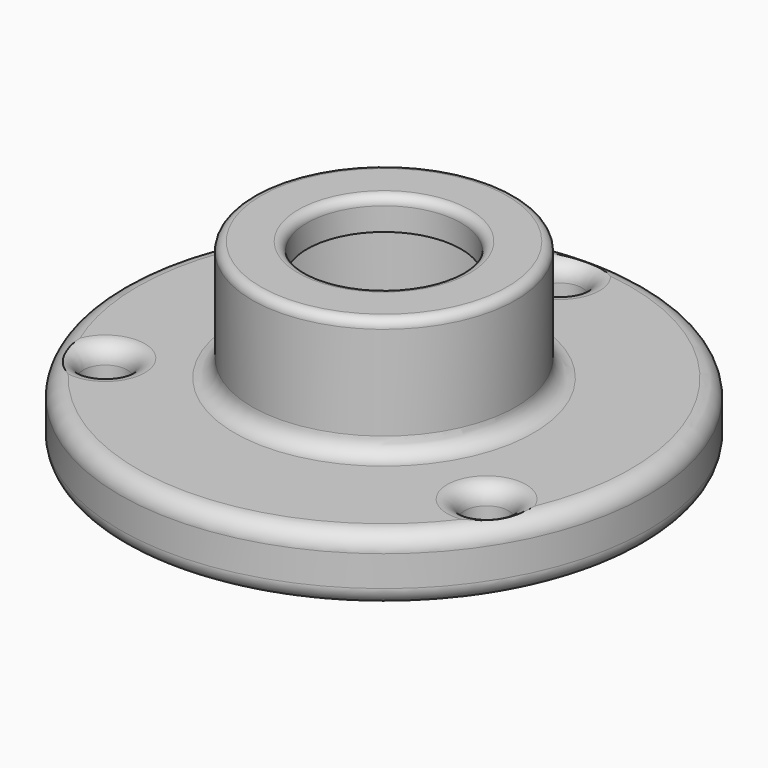
from build123d import *

# Parameters (mm, degrees)
F0_W     = 38.1
F0_H     = 34.6730154096
F2_R     = 6.35
F3_DEPTH = 18.9502071143
F4_R     = 31.75
F5_DEPTH = 44.45
F6_R     = 22.225
F7_DEPTH = 25.4
F8_R     = 2.54


# Not quite as in the source:
# - a fillet or chamfer that OpenCascade refuses, or shapes differently, is made with other operations: its cross-section is extruded or revolved along the edge and cut away or added


with BuildPart() as f1:
    # F0 (on Front) → F1 (revolve)
    with BuildSketch(Plane.XZ):
        Polygon((-76.2, 0), (0, 0), (0, 18.9492071143), (-38.1, 18.9492071143), (-76.2, 18.9492071143), align=None)
        with Locations((-19.05, 36.2857148192)):
            Rectangle(F0_W, F0_H)
    revolve(axis=Axis((0, 0, 36.2857148192), (0, 0, -1)))

    # F2 (on face) → F3 (cut, through all)
    with BuildSketch(Plane.XY.offset(18.9492071143)):
        with Locations((-54.9926131403, -31.75)):
            Circle(F2_R)
        with Locations((54.9926131403, -31.75)):
            Circle(F2_R)
        with Locations((0, 63.5)):
            Circle(F2_R)
    extrude(amount=-F3_DEPTH, mode=Mode.SUBTRACT)

    # F4 (on face) → F5 (cut)
    with BuildSketch(Plane(origin=(0, 0, 0), x_dir=(1, 0, 0), z_dir=(0, 0, -1))):
        Circle(F4_R)
    extrude(amount=-F5_DEPTH, mode=Mode.SUBTRACT)

    # F6 (on face) → F7 (cut)
    with BuildSketch(Plane.XY.offset(53.622222524)):
        Circle(F6_R)
    extrude(amount=-F7_DEPTH, mode=Mode.SUBTRACT)

    # F8
    f8_edges = [f1.edges().sort_by_distance(p)[0] for p in [
        (38.1, 0, 53.622223),
        (-22.225, 0, 53.622223),
    ]]
    fillet(f8_edges, radius=F8_R)

    # F9: fillet of radius 5.08 on 5 edges, made by hand

    # F9_s1 → F9_t2 (revolve)
    with BuildSketch(Plane.XZ):
        with BuildLine():
            ThreePointArc((-38.0996, 24.0301727998), (-39.5878975516, 20.4371046659), (-43.1809656854, 18.9488071143))
            Line((-43.1809656854, 18.9488071143), (-43.1809656854, 18.4406705458))
            ThreePointArc((-43.1809656854, 18.4406705458), (-40.6404828427, 18.4410705458), (-38.1, 18.4410705458))
            Line((-38.1, 18.4410705458), (-37.5918634315, 18.9492071143))
            ThreePointArc((-37.5918634315, 18.9492071143), (-37.5918634315, 21.489689957), (-37.5914634315, 24.0301727998))
            Line((-37.5914634315, 24.0301727998), (-38.0996, 24.0301727998))
        make_face()
    revolve(axis=Axis((0, 0, 18.9492071143), (0, 0, -1)))

    # F9_s3 → F9_t4 (revolve, cut)
    with BuildSketch(Plane.XZ):
        with BuildLine():
            ThreePointArc((-71.1190343146, 18.9496071143), (-74.7121024484, 17.4613095628), (-76.2004, 13.8682414289))
            Line((-76.2004, 13.8682414289), (-76.7085365685, 13.8682414289))
            ThreePointArc((-76.7085365685, 13.8682414289), (-76.7081365685, 16.4087242716), (-76.7081365685, 18.9492071143))
            Line((-76.7081365685, 18.9492071143), (-76.2, 19.4573436829))
            ThreePointArc((-76.2, 19.4573436829), (-73.6595171573, 19.4573436829), (-71.1190343146, 19.4577436829))
            Line((-71.1190343146, 19.4577436829), (-71.1190343146, 18.9496071143))
        make_face()
    revolve(axis=Axis((0, 0, 18.9492071143), (0, 0, -1)), mode=Mode.SUBTRACT)

    # F9_s5 → F9_t6 (revolve, cut)
    with BuildSketch(Plane.XZ.offset(31.75)):
        with BuildLine():
            ThreePointArc((-43.5616474549, 18.9496071143), (-47.1547155887, 17.4613095628), (-48.6430131403, 13.8682414289))
            Line((-48.6430131403, 13.8682414289), (-49.1511497089, 13.8682414289))
            ThreePointArc((-49.1511497089, 13.8682414289), (-49.1507497089, 16.4087242716), (-49.1507497089, 18.9492071143))
            Line((-49.1507497089, 18.9492071143), (-48.6426131403, 19.4573436829))
            ThreePointArc((-48.6426131403, 19.4573436829), (-46.1021302976, 19.4573436829), (-43.5616474549, 19.4577436829))
            Line((-43.5616474549, 19.4577436829), (-43.5616474549, 18.9496071143))
        make_face()
    revolve(axis=Axis((-54.9926131403, -31.75, 18.9492071143), (0, 0, 1)), mode=Mode.SUBTRACT)

    # F9_s7 → F9_t8 (revolve, cut)
    with BuildSketch(Plane.XZ.offset(31.75)):
        with BuildLine():
            ThreePointArc((66.4235788257, 18.9496071143), (62.8305106919, 17.4613095628), (61.3422131403, 13.8682414289))
            Line((61.3422131403, 13.8682414289), (60.8340765718, 13.8682414289))
            ThreePointArc((60.8340765718, 13.8682414289), (60.8344765718, 16.4087242716), (60.8344765718, 18.9492071143))
            Line((60.8344765718, 18.9492071143), (61.3426131403, 19.4573436829))
            ThreePointArc((61.3426131403, 19.4573436829), (63.883095983, 19.4573436829), (66.4235788257, 19.4577436829))
            Line((66.4235788257, 19.4577436829), (66.4235788257, 18.9496071143))
        make_face()
    revolve(axis=Axis((54.9926131403, -31.75, 18.9492071143), (0, 0, 1)), mode=Mode.SUBTRACT)

    # F9_s9 → F9_t10 (revolve, cut)
    with BuildSketch(Plane.XZ.offset(-63.5)):
        with BuildLine():
            ThreePointArc((11.4309656854, 18.9496071143), (7.8378975516, 17.4613095628), (6.3496, 13.8682414289))
            Line((6.3496, 13.8682414289), (5.8414634315, 13.8682414289))
            ThreePointArc((5.8414634315, 13.8682414289), (5.8418634315, 16.4087242716), (5.8418634315, 18.9492071143))
            Line((5.8418634315, 18.9492071143), (6.35, 19.4573436829))
            ThreePointArc((6.35, 19.4573436829), (8.8904828427, 19.4573436829), (11.4309656854, 19.4577436829))
            Line((11.4309656854, 19.4577436829), (11.4309656854, 18.9496071143))
        make_face()
    revolve(axis=Axis((0, 63.5, 18.9492071143), (0, 0, 1)), mode=Mode.SUBTRACT)

    # F10: fillet of radius 5.08 on 5 edges, made by hand

    # F10_s1 → F10_t2 (revolve, cut)
    with BuildSketch(Plane.XZ):
        with BuildLine():
            ThreePointArc((-76.2, 5.08), (-74.7121024484, 1.4878975516), (-71.12, 0))
            Line((-71.12, 0), (-76.2, 0))
            Line((-76.2, 0), (-76.2, 5.08))
        make_face()
    revolve(axis=Axis((0, 0, 0), (0, 0, -1)), mode=Mode.SUBTRACT)

    # F10_s3 → F10_t4 (revolve, cut)
    with BuildSketch(Plane.XZ.offset(31.75)):
        with BuildLine():
            ThreePointArc((61.3426131403, 5.08), (62.8305106919, 1.4878975516), (66.4226131403, 0))
            Line((66.4226131403, 0), (61.3426131403, 0))
            Line((61.3426131403, 0), (61.3426131403, 5.08))
        make_face()
    revolve(axis=Axis((54.9926131403, -31.75, 0), (0, 0, 1)), mode=Mode.SUBTRACT)

    # F10_s5 → F10_t6 (revolve, cut)
    with BuildSketch(Plane.XZ):
        with BuildLine():
            ThreePointArc((36.83, 0), (33.2378975516, 1.4878975516), (31.75, 5.08))
            Line((31.75, 5.08), (31.75, 0))
            Line((31.75, 0), (36.83, 0))
        make_face()
    revolve(axis=Axis((0, 0, 0), (0, 0, -1)), mode=Mode.SUBTRACT)

    # F10_s7 → F10_t8 (revolve, cut)
    with BuildSketch(Plane.XZ.offset(31.75)):
        with BuildLine():
            ThreePointArc((-48.6426131403, 5.08), (-47.1547155887, 1.4878975516), (-43.5626131403, 0))
            Line((-43.5626131403, 0), (-48.6426131403, 0))
            Line((-48.6426131403, 0), (-48.6426131403, 5.08))
        make_face()
    revolve(axis=Axis((-54.9926131403, -31.75, 0), (0, 0, 1)), mode=Mode.SUBTRACT)

    # F10_s9 → F10_t10 (revolve, cut)
    with BuildSketch(Plane.XZ.offset(-63.5)):
        with BuildLine():
            ThreePointArc((6.35, 5.08), (7.8378975516, 1.4878975516), (11.43, 0))
            Line((11.43, 0), (6.35, 0))
            Line((6.35, 0), (6.35, 5.08))
        make_face()
    revolve(axis=Axis((0, 63.5, 0), (0, 0, 1)), mode=Mode.SUBTRACT)


solid = f1.part
